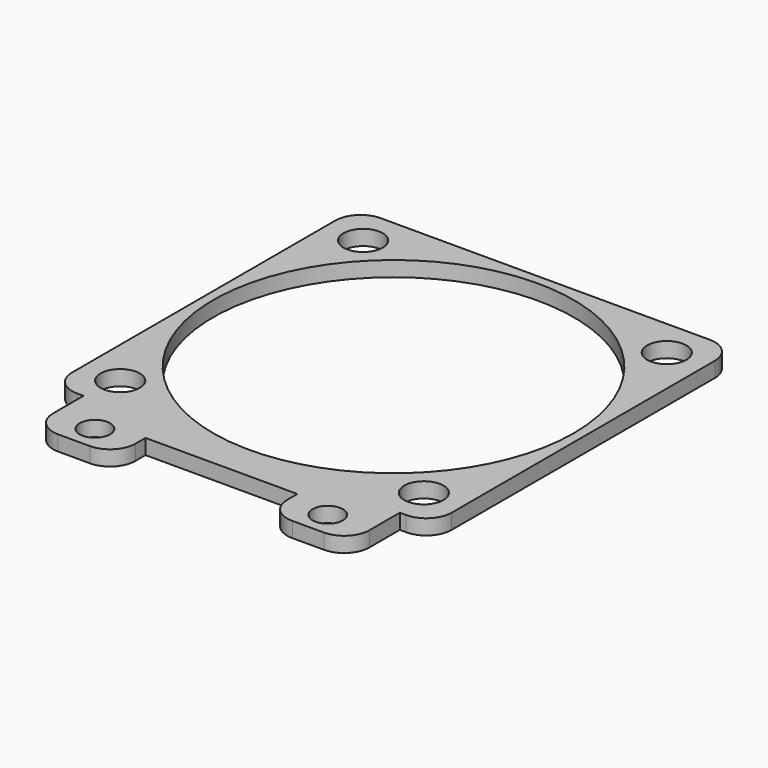
from build123d import *

# Parameters (mm, degrees)
F0_R     = 1.55
F0_R_2   = 14.25
F0_R_3   = 1.2
F0_W     = 12
F0_H     = 2
F1_DEPTH = 1.2
F2_R     = 2


with BuildPart() as f1:
    # F0 (on Top) → F1 (new body)
    with BuildSketch(Plane.XY):
        Polygon((12.5, -15), (15, -15), (15, 15), (-15, 15), (-15, -15), (-12.5, -15), (-6, -15), (6, -15), align=None)
        with Locations((-12, -12)):
            Circle(F0_R, mode=Mode.SUBTRACT)
        with Locations((12, -12)):
            Circle(F0_R, mode=Mode.SUBTRACT)
        with Locations((-12, 12)):
            Circle(F0_R, mode=Mode.SUBTRACT)
        Circle(F0_R_2, mode=Mode.SUBTRACT)
        with Locations((12, 12)):
            Circle(F0_R, mode=Mode.SUBTRACT)
        Polygon((-6, -17), (-6, -15), (-12.5, -15), (-12.5, -20), (-6, -20), align=None)
        with Locations((-9.2, -18)):
            Circle(F0_R_3, mode=Mode.SUBTRACT)
        with Locations((0, -16)):
            Rectangle(F0_W, F0_H)
        Polygon((12.5, -20), (12.5, -15), (6, -15), (6, -17), (6, -20), align=None)
        with Locations((9.2, -18)):
            Circle(F0_R_3, mode=Mode.SUBTRACT)
    extrude(amount=F1_DEPTH)

    # F2
    f2_edges = [f1.edges().sort_by_distance(p)[0] for p in [
        (15, -15, 0.6),
        (-15, -15, 0.6),
        (-15, 15, 0.6),
        (15, 15, 0.6),
        (-12.5, -20, 0.6),
        (-6, -20, 0.6),
        (6, -20, 0.6),
        (12.5, -20, 0.6),
    ]]
    fillet(f2_edges, radius=F2_R)


solid = f1.part
